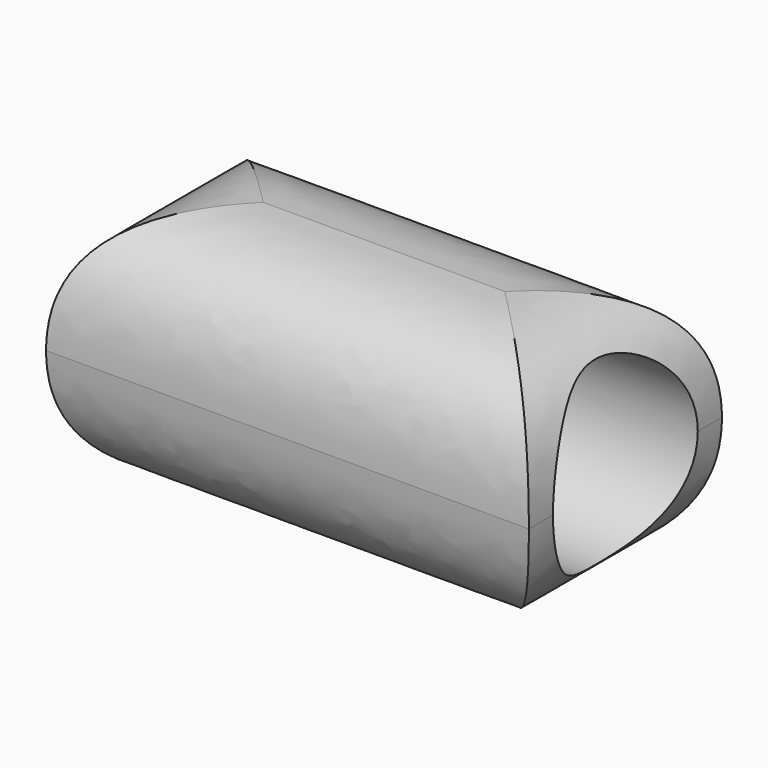
from build123d import *

# Parameters (mm, degrees)
F0_W          = 101.6
F0_H          = 50.8
F1_DEPTH      = 25.4
F2_T1_DEPTH   = 177.8
F2_T3_DEPTH   = 228.6
F4_R          = 19.05
F5_DEPTH      = 50.8
F5_DEPTH_BACK = 50.8


# Not quite as in the source:
# - a fillet or chamfer that OpenCascade refuses, or shapes differently, is made with other operations: its cross-section is extruded or revolved along the edge and cut away or added
# - the program builds the solid bodies; features that only make, move or delete a surface that nothing else refers to are left out


with BuildPart() as f1:
    # F0 (on Top) → F1 (new body)
    with BuildSketch(Plane.XY):
        Rectangle(F0_W, F0_H)
    extrude(amount=F1_DEPTH)

    # F2: fillet of radius 25.4 on 4 edges, made by hand

    # F2_s2 → F2_t1 (cut)
    with BuildSketch(Plane.XZ.offset(-88.9)):
        with BuildLine():
            add(Edge.make_bspline(
                [(50.8, 0), (50.8, 25.4), (25.4, 25.4)],
                knots=[0, 0, 0, 1, 1, 1], degree=2, weights=[1, 1, 1]))
            Line((25.4, 25.4), (50.8, 25.4))
            Line((50.8, 25.4), (50.8, 0))
        make_face()
        with BuildLine():
            add(Edge.make_bspline(
                [(-50.8, 0), (-50.8, 25.4), (-25.4, 25.4)],
                knots=[0, 0, 0, 1, 1, 1], degree=2, weights=[1, 1, 1]))
            Line((-25.4, 25.4), (-50.8, 25.4))
            Line((-50.8, 25.4), (-50.8, 0))
        make_face()
    extrude(amount=F2_T1_DEPTH, mode=Mode.SUBTRACT)

    # F2_s4 → F2_t3 (cut)
    with BuildSketch(Plane.YZ.offset(-114.3)):
        with BuildLine():
            add(Edge.make_bspline(
                [(25.4, 0), (25.4, 25.4), (0, 25.4)],
                knots=[0, 0, 0, 1, 1, 1], degree=2, weights=[1, 1, 1]))
            Line((0, 25.4), (25.4, 25.4))
            Line((25.4, 25.4), (25.4, 0))
        make_face()
        with BuildLine():
            add(Edge.make_bspline(
                [(-25.4, 0), (-25.4, 25.4), (0, 25.4)],
                knots=[0, 0, 0, 1, 1, 1], degree=2, weights=[1, 1, 1]))
            Line((0, 25.4), (-25.4, 25.4))
            Line((-25.4, 25.4), (-25.4, 0))
        make_face()
    extrude(amount=F2_T3_DEPTH, mode=Mode.SUBTRACT)

    # F3: F1 across plane


with BuildPart() as f1_1:
    add(f1.part)
    add(f1.part.mirror(Plane.XY))

    # F4 (on Right) → F5 (cut, two sides)
    with BuildSketch(Plane.YZ) as f5_sk:
        Circle(F4_R)
    extrude(amount=-F5_DEPTH, mode=Mode.SUBTRACT)
    extrude(f5_sk.sketch, amount=F5_DEPTH_BACK, mode=Mode.SUBTRACT)


solid = f1_1.part
